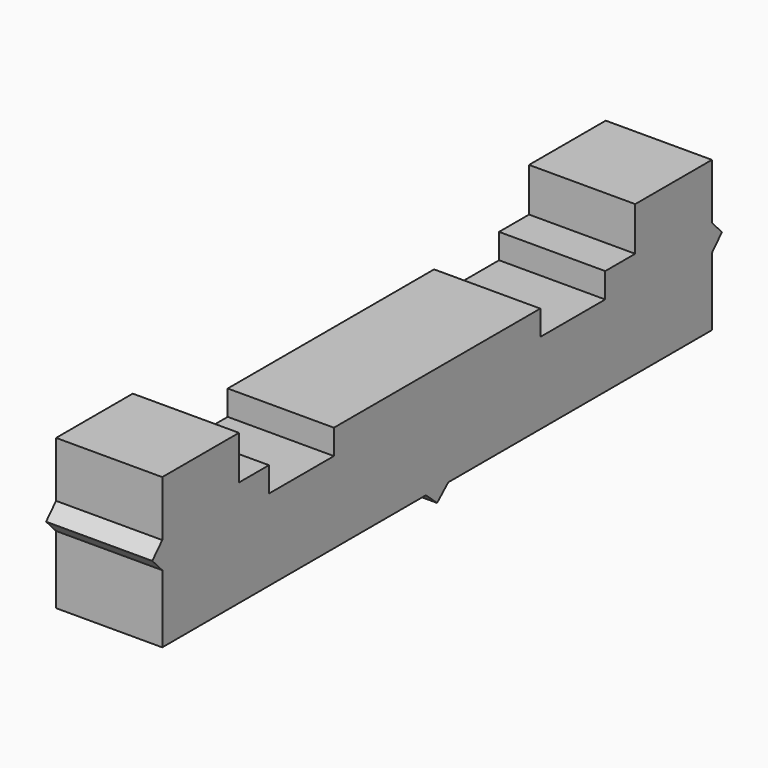
from build123d import *

# Parameters (mm, degrees)
F1_DEPTH = 17
F3_DEPTH = 17
F5_DEPTH = 17


# Not quite as in the source:
# - a pattern or mirror of a feature is missing from the dataset's text; its kind, count and spacing are read off the source's solid


with BuildPart() as f1:
    # F0 (on Right) → F1 (new body)
    with BuildSketch(Plane.YZ):
        Polygon((0, 24), (0, 0), (110, 0), (110, 24), (94.65, 24), (94.65, 17), (88.65, 17), (88.65, 13), (75.65, 13), (75.65, 17), (34.35, 17), (34.35, 13), (21.35, 13), (21.35, 17), (15.35, 17), (15.35, 24), align=None)
    extrude(amount=F1_DEPTH)

    # F2 (on face) → F3 (join, through all)
    with BuildSketch(Plane.YZ.offset(17)):
        Polygon((57.2362883389, 0), (55, 0), (55, -2), align=None)
        Polygon((55, 0), (52.7637116611, 0), (55, -2), align=None)
    extrude(amount=-F3_DEPTH)

    # F4 (on face) → F5 (join, through all)
    with BuildSketch(Plane.YZ.offset(17)):
        Polygon((0, 10.8757078871), (0, 13), (-2, 13), align=None)
        Polygon((-2, 13), (0, 13), (0, 15.1242921129), align=None)
    f5 = extrude(amount=-F5_DEPTH)

    # F5_copies: F5 across plane
    add(f5.mirror(Plane.ZX.offset(55)))


solid = f1.part
